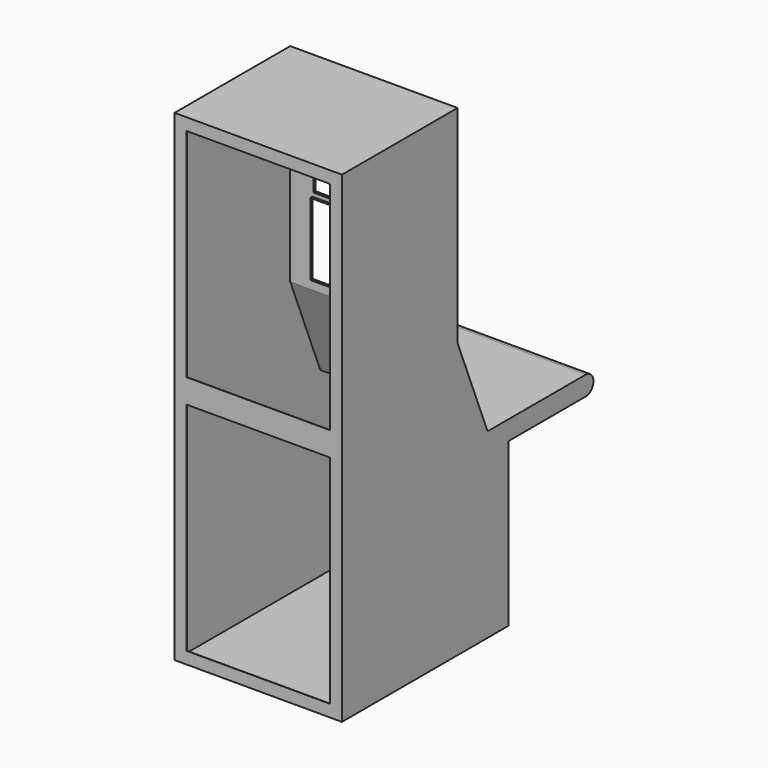
from build123d import *

# Parameters (mm, degrees)
F1_DEPTH = 695
F2_W     = 595
F2_H     = 900
F3_DEPTH = 1.2
F4_W     = 509
F4_H     = 299
F5_DEPTH = 10
F4_W_2   = 465
F4_H_2   = 431
F4_W_3   = 10
F6_DEPTH = 10
F7_W     = 465
F7_H     = 605
F7_W_2   = 10
F8_DEPTH = 10
F9_T     = -1.2


# Not quite as in the source:
# - a shell that OpenCascade refuses in one call is made with other operations: the cavity is built on its own and cut out


with BuildPart() as f1:
    # F0 (on Right) → F1 (new body)
    with BuildSketch(Plane.YZ):
        with BuildLine():
            Line((0, 2000), (0, 0))
            Line((0, 0), (865, 0))
            Line((865, 0), (865, 675))
            Line((865, 675), (1265, 675))
            ThreePointArc((1265, 675), (1305, 715), (1265, 755))
            Line((1265, 755), (755.5500969465, 755))
            Line((755.5500969465, 755), (600, 1140))
            Line((600, 1140), (600, 2000))
            Line((600, 2000), (0, 2000))
        make_face()
    extrude(amount=-F1_DEPTH)

    # F2 (on face) → F3 (cut)
    with BuildSketch(Plane.XZ):
        with Locations((-347.5, 1500)):
            Rectangle(F2_W, F2_H)
        with Locations((-347.5, 500)):
            Rectangle(F2_W, F2_H)
    extrude(amount=-F3_DEPTH, mode=Mode.SUBTRACT)

    # F4 (on face) → F5 (cut)
    with BuildSketch(Plane(origin=(0, 600, 0), x_dir=(-1, 0, 0), z_dir=(0, 1, 0))):
        with Locations((347.5, 1329.5)):
            Rectangle(F4_W, F4_H)
    extrude(amount=-F5_DEPTH, mode=Mode.SUBTRACT)

    # F4 (on face) → F6 (cut)
    with BuildSketch(Plane(origin=(0, 600, 0), x_dir=(-1, 0, 0), z_dir=(0, 1, 0))):
        with Locations((347.5, 1719.5)):
            Rectangle(F4_W_2, F4_H_2)
        with Locations((110, 1719.5)):
            Rectangle(F4_W_3, F4_H_2)
        with Locations((585, 1719.5)):
            Rectangle(F4_W_3, F4_H_2)
    extrude(amount=-F6_DEPTH, mode=Mode.SUBTRACT)

    # F7 (on face) → F8 (cut)
    with BuildSketch(Plane(origin=(0, 865, 0), x_dir=(-1, 0, 0), z_dir=(0, 1, 0))):
        with Locations((347.5, 352.5)):
            Rectangle(F7_W, F7_H)
        with Locations((110, 352.5)):
            Rectangle(F7_W_2, F7_H)
        with Locations((585, 352.5)):
            Rectangle(F7_W_2, F7_H)
    extrude(amount=-F8_DEPTH, mode=Mode.SUBTRACT)

    # F9: a shell. OpenCascade refuses it in one call, so the cavity is built on its own and cut out:
    # the body offset inwards by the wall thickness, plus a prism from it out through each open face.
    f9_core = offset(f1.part, amount=F9_T, kind=Kind.INTERSECTION, mode=Mode.PRIVATE)
    f9_exits = [f9_core.faces().sort_by_distance(p)[0] for p in [
        (-347.5, 588.8, 1719.5),
        (-347.5, 588.8, 1329.5),
        (-347.5, 853.8, 352.5),
        (-347.5, 2.4, 500),
        (-347.5, 2.4, 1500),
    ]]
    add(f9_core, mode=Mode.SUBTRACT)
    extrude(f9_exits, amount=-F9_T, mode=Mode.SUBTRACT)


solid = f1.part
